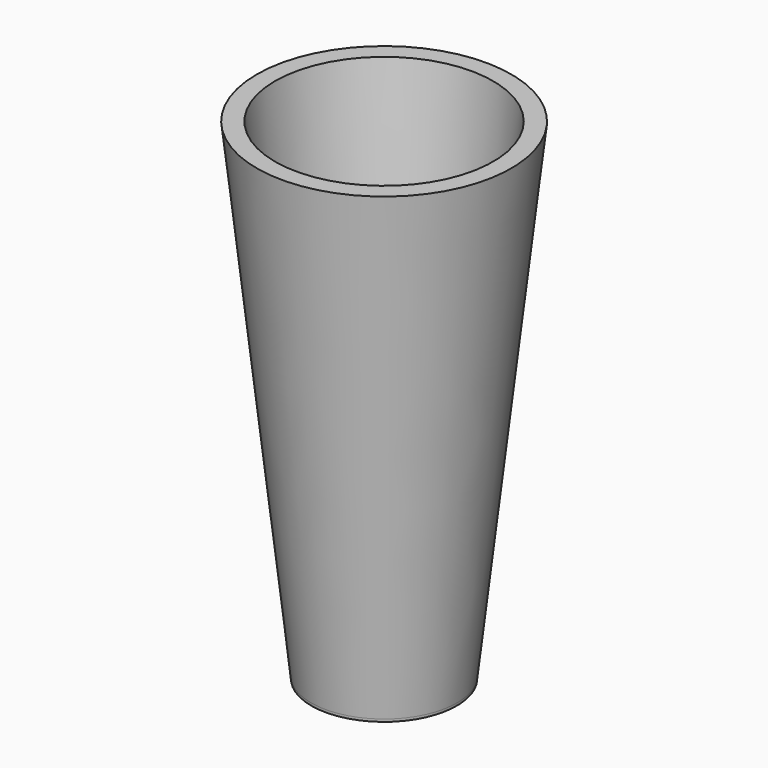
from build123d import *

# Parameters (mm, degrees)
F0_W = 0.635
F0_H = 0.9395605023


with BuildPart() as f1:
    # F0 (on Front) → F1 (revolve)
    with BuildSketch(Plane.XZ):
        Polygon((-19.05, -94.2954702053), (-19.1543956114, -93.355909703), (-25.5043956114, -93.355909703), (-25.4, -94.2954702053), align=None)
        with Locations((-13.0175, -93.8256899541)):
            Rectangle(F0_W, F0_H)
        Polygon((0, -68.8954702053), (0, -68.2604702053), (-13.335, -68.2604702053), (-13.335, -93.355909703), (-12.7, -93.355909703), (-12.7, -68.8954702053), align=None)
        Polygon((-13.335, -93.355909703), (-19.1543956114, -93.355909703), (-19.05, -94.2954702053), (-13.335, -94.2954702053), align=None)
        Polygon((-19.1543956114, -93.355909703), (-38.1, 77.1545297947), (-44.45, 77.1545297947), (-25.5043956114, -93.355909703), align=None)
    revolve(axis=Axis((0, 0, 4.1295297947), (0, 0, 1)))


solid = f1.part
